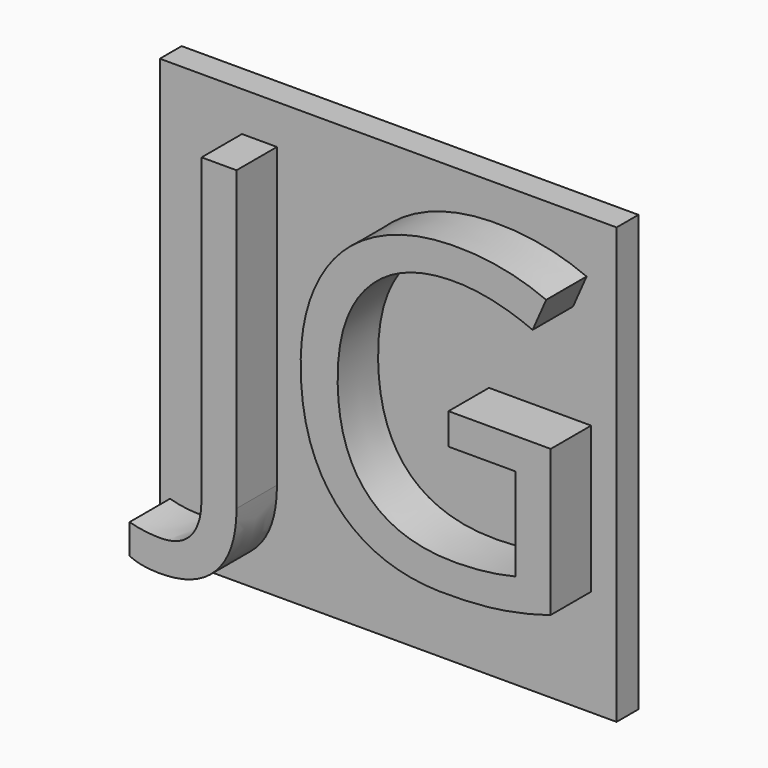
from build123d import *

# Parameters (mm, degrees)
F0_TEXT_SIZE = 105.8333333333
F1_DEPTH     = 12.7
F2_W         = 114.7839650512
F2_H         = 109.4034612179
F3_DEPTH     = 6.858


# Not quite as in the source:
# - Text() gives the source's letters only with a copy of the font that has no kerning and outlines rounded to 1/6400 em; it was checked with that copy


with BuildPart() as f1:
    # F0 (on Front) → F1 (new body)
    with BuildSketch(Plane.XZ):
        with Locations((-55.1316210848, -37.7207129756)):
            Text('JG', F0_TEXT_SIZE, font='Open Sans', text_align=(TextAlign.LEFT, TextAlign.BOTTOM))
    extrude(amount=F1_DEPTH)

    # F2 (on Front) → F3 (join)
    with BuildSketch(Plane.XZ):
        with Locations((-8.5661746562, -6.9140195847)):
            Rectangle(F2_W, F2_H)
    extrude(amount=-F3_DEPTH)


solid = f1.part
